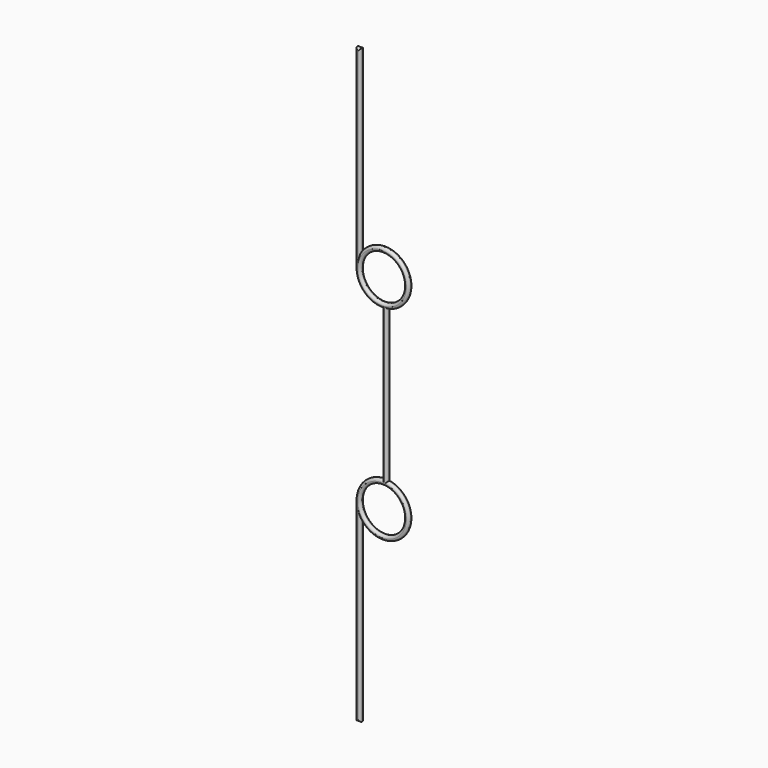
from build123d import *

# Parameters (mm, degrees)
F0_R     = 4.4999999525
F1_DEPTH = 1
F3_R     = 0.49999


# Not quite as in the source:
# - a fillet or chamfer is up to 0.001 mm smaller than in the source, because OpenCascade refuses the exact size


with BuildPart() as f1:
    # F0 (on Front) → F1 (new body)
    with BuildSketch(Plane.XZ):
        with BuildLine():
            Line((0, 40), (0, 0))
            Line((0, 0), (1, 0))
            Line((1, 0), (1, 36.8377223398))
            ThreePointArc((1, 36.8377223398), (10.1288568078, 37.0295312402), (6.5000001341, 45.4083268884))
            Line((6.5000001341, 45.4083268884), (6.5000001341, 61.0393770039))
            Line((6.5000001341, 61.0393770039), (5.5, 61.0393770039))
            Line((5.5, 61.0393770039), (5.5, 45.5))
            ThreePointArc((5.5, 45.5), (1.6109127035, 43.8890872965), (0, 40))
        make_face()
        with Locations((5.5, 40)):
            Circle(F0_R, mode=Mode.SUBTRACT)
    extrude(amount=F1_DEPTH)

    # F2: F1 across face


with BuildPart() as f1_1:
    add(f1.part)
    add(f1.part.mirror(Plane(origin=(6.0000000671, -0.5, 61.0393770039), x_dir=(1, 0, 0), z_dir=(0, 0, 1))))

    # F3 (radius 0.5 in the source; OpenCascade refuses exactly that, so slightly less here)
    f3_edges = [f1_1.edges().sort_by_distance(p)[0] for p in [
        (6.5, -1, 61.039377),
        (10.128857, -1, 85.049223),
        (1, -1, 103.659893),
        (0.5, -1, 122.078754),
        (0, -1, 102.078754),
        (1.610913, -1, 78.189667),
        (5.5, -1, 61.039377),
        (1.610913, -1, 43.889087),
        (0, -1, 20),
        (0.5, -1, 0),
        (1, -1, 18.418861),
        (10.128857, -1, 37.029531),
        (1, -1, 40),
        (1, -1, 82.078754),
        (6.5, 0, 61.039377),
        (10.128857, 0, 85.049223),
        (1, 0, 103.659893),
        (0.5, 0, 122.078754),
        (0, 0, 102.078754),
        (1.610913, 0, 78.189667),
        (5.5, 0, 61.039377),
        (1.610913, 0, 43.889087),
        (0, 0, 20),
        (0.5, 0, 0),
        (1, 0, 18.418861),
        (10.128857, 0, 37.029531),
        (1, 0, 40),
        (1, 0, 82.078754),
    ]]
    fillet(f3_edges, radius=F3_R)


solid = f1_1.part
